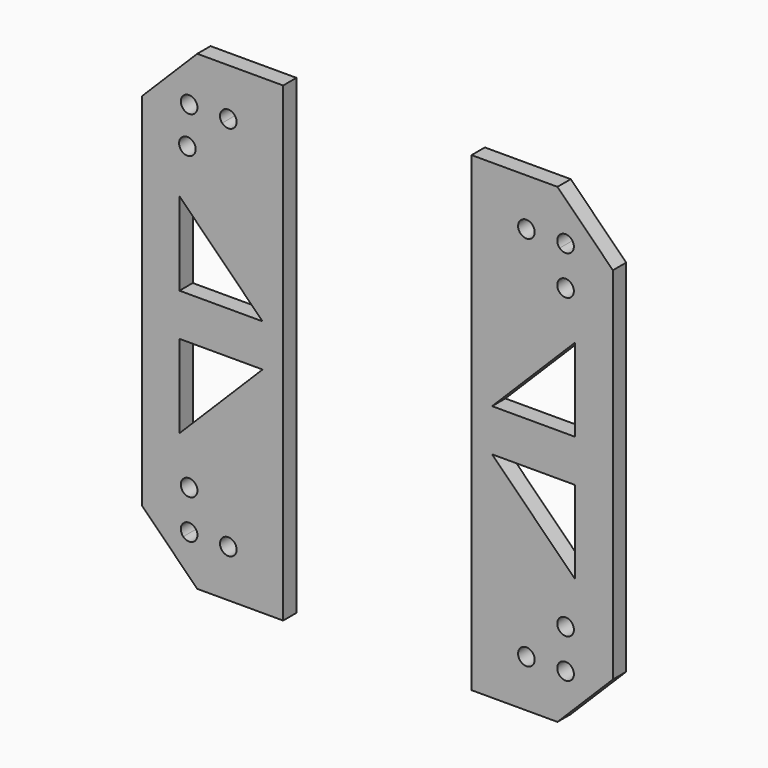
from build123d import *

# Parameters (mm, degrees)
F0_R      = 1.5
F1_DEPTH  = 3
F2_SIZE   = 10
F2_2_SIZE = 10


with BuildPart() as f1:
    # F0 (on Front) → F1 (new body)
    with BuildSketch(Plane.XZ):
        Polygon((42.5, 32.5), (42.5, 42.5), (37.5, 37.5), align=None)
        Polygon((37.5, 37.5), (42.5, 42.5), (32.5, 42.5), align=None)
        Polygon((42.5, -32.5), (42.5, 32.5), (37.5, 37.5), (32.5, 42.5), (17, 42.5), (17, -42.5), (32.5, -42.5), (37.5, -37.5), align=None)
        with Locations((26.8933982822, -33.9644660941)):
            Circle(F0_R, mode=Mode.SUBTRACT)
        with BuildLine():
            ThreePointArc((35.4644660941, -33.9644660941), (35.3502853928, -34.5384912426), (35.0251262658, -35.0251262658))
            ThreePointArc((35.0251262658, -35.0251262658), (32.9038059223, -35.0251262658), (32.9038059223, -32.9038059223))
            ThreePointArc((32.9038059223, -32.9038059223), (34.5384912426, -32.5786467953), (35.4644660941, -33.9644660941))
        make_face(mode=Mode.SUBTRACT)
        with Locations((33.9644660941, -26.8933982822)):
            Circle(F0_R, mode=Mode.SUBTRACT)
        Polygon((20.7055291533, -3.823871389), (35.7055291533, -3.823871389), (35.7055291533, -18.823871389), align=None, mode=Mode.SUBTRACT)
        Polygon((35.7055291533, 3.823871389), (20.7055291533, 3.823871389), (35.7055291533, 18.823871389), align=None, mode=Mode.SUBTRACT)
        with BuildLine():
            ThreePointArc((35.4644660941, 26.8933982822), (33.3904409455, 25.5075789834), (32.9038059223, 27.954058454))
            ThreePointArc((32.9038059223, 27.954058454), (34.5384912426, 28.279217581), (35.4644660941, 26.8933982822))
        make_face(mode=Mode.SUBTRACT)
        with BuildLine():
            ThreePointArc((28.3933982822, 33.9644660941), (28.279217581, 33.3904409455), (27.954058454, 32.9038059223))
            ThreePointArc((27.954058454, 32.9038059223), (25.5075789834, 34.5384912426), (28.3933982822, 33.9644660941))
        make_face(mode=Mode.SUBTRACT)
        with BuildLine():
            ThreePointArc((32.9038059223, 32.9038059223), (32.9038059223, 35.0251262658), (35.0251262658, 35.0251262658))
            ThreePointArc((35.0251262658, 35.0251262658), (35.3502853928, 34.5384912426), (35.4644660941, 33.9644660941))
            ThreePointArc((35.4644660941, 33.9644660941), (34.5384912426, 32.5786467953), (32.9038059223, 32.9038059223))
        make_face(mode=Mode.SUBTRACT)
        Polygon((42.5, -42.5), (42.5, -32.5), (37.5, -37.5), align=None)
        Polygon((32.5, -42.5), (42.5, -42.5), (37.5, -37.5), align=None)
    extrude(amount=F1_DEPTH)

    # F2
    f2_edges = [f1.edges().sort_by_distance(p)[0] for p in [
        (42.5, -1.5, 42.5),
        (42.5, -1.5, -42.5),
    ]]
    chamfer(f2_edges, length=F2_SIZE)


with BuildPart() as f1b:
    # F0 (on Front) → F1, piece 2 (new body)
    with BuildSketch(Plane.XZ):
        Polygon((-37.5, 37.5), (-42.5, 42.5), (-42.5, 32.5), align=None)
        Polygon((-32.5, 42.5), (-42.5, 42.5), (-37.5, 37.5), align=None)
        Polygon((-37.5, 37.5), (-42.5, 32.5), (-42.5, -32.5), (-37.5, -37.5), (-32.5, -42.5), (-17, -42.5), (-17, 42.5), (-32.5, 42.5), align=None)
        with BuildLine():
            ThreePointArc((-32.4644660941, -33.9644660941), (-33.3904409455, -35.3502853928), (-35.0251262658, -35.0251262658))
            ThreePointArc((-35.0251262658, -35.0251262658), (-35.0251262658, -32.9038059223), (-32.9038059223, -32.9038059223))
            ThreePointArc((-32.9038059223, -32.9038059223), (-32.5786467953, -33.3904409455), (-32.4644660941, -33.9644660941))
        make_face(mode=Mode.SUBTRACT)
        with Locations((-26.8933982822, -33.9644660941)):
            Circle(F0_R, mode=Mode.SUBTRACT)
        with Locations((-33.9644660941, -26.8933982822)):
            Circle(F0_R, mode=Mode.SUBTRACT)
        Polygon((-20.7055291533, -3.823871389), (-35.7055291533, -18.823871389), (-35.7055291533, -3.823871389), align=None, mode=Mode.SUBTRACT)
        Polygon((-35.7055291533, 3.823871389), (-35.7055291533, 18.823871389), (-20.7055291533, 3.823871389), align=None, mode=Mode.SUBTRACT)
        with BuildLine():
            ThreePointArc((-32.7795228992, 27.2231633162), (-35.6780717969, 26.6808894181), (-33.1716042066, 28.2343587329))
            ThreePointArc((-33.1716042066, 28.2343587329), (-32.8809740014, 27.7654372144), (-32.7795228992, 27.2231633162))
        make_face(mode=Mode.SUBTRACT)
        with BuildLine():
            ThreePointArc((-32.9038059223, 32.9038059223), (-35.0251262658, 32.9038059223), (-35.0251262658, 35.0251262658))
            ThreePointArc((-35.0251262658, 35.0251262658), (-33.3904409455, 35.3502853928), (-32.4644660941, 33.9644660941))
            ThreePointArc((-32.4644660941, 33.9644660941), (-32.5786467953, 33.3904409455), (-32.9038059223, 32.9038059223))
        make_face(mode=Mode.SUBTRACT)
        with BuildLine():
            ThreePointArc((-25.3933982822, 33.9644660941), (-26.3511243841, 32.5659171963), (-28.0013169747, 32.9532706774))
            ThreePointArc((-28.0013169747, 32.9532706774), (-27.4356721803, 35.3630149918), (-25.3933982822, 33.9644660941))
        make_face(mode=Mode.SUBTRACT)
        Polygon((-37.5, -37.5), (-42.5, -32.5), (-42.5, -42.5), align=None)
        Polygon((-37.5, -37.5), (-42.5, -42.5), (-32.5, -42.5), align=None)
    extrude(amount=F1_DEPTH)

    # F2#2
    f2_2_edges = [f1b.edges().sort_by_distance(p)[0] for p in [
        (-42.5, -1.5, 42.5),
        (-42.5, -1.5, -42.5),
    ]]
    chamfer(f2_2_edges, length=F2_2_SIZE)


solid = Compound([f1.part, f1b.part])
